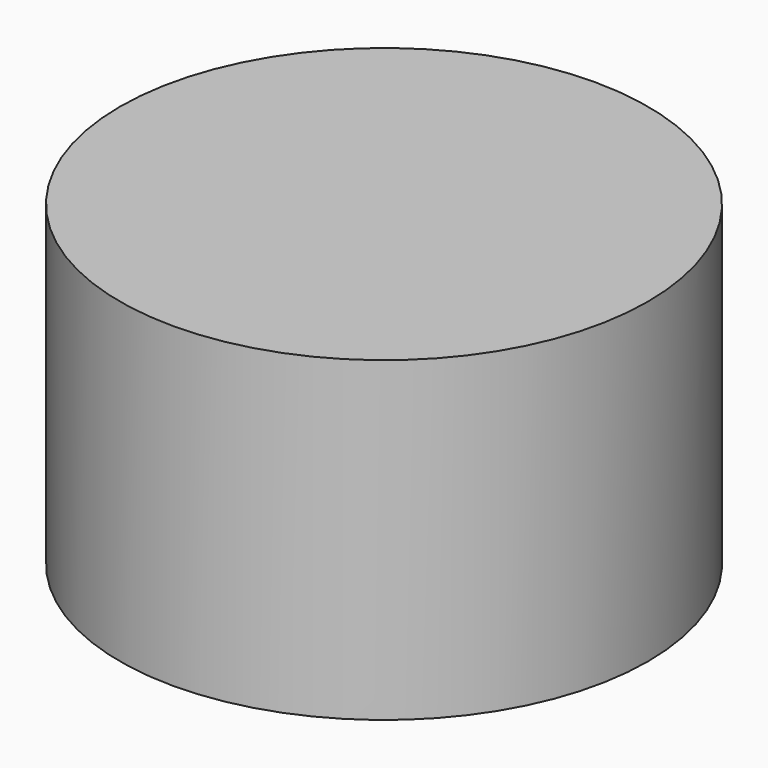
from build123d import *

# Parameters (mm, degrees)
F0_W = 250
F0_H = 300


# Not quite as in the source:
# - a feature of the source that left no trace in its solid (it failed there, or was rolled back) is left out


with BuildPart() as f1:
    # F0 (on Front) → F1 (revolve)
    with BuildSketch(Plane.XZ):
        with Locations((125, 150)):
            Rectangle(F0_W, F0_H)
    revolve(axis=Axis((0, 0, 150), (0, 0, 1)))


solid = f1.part
